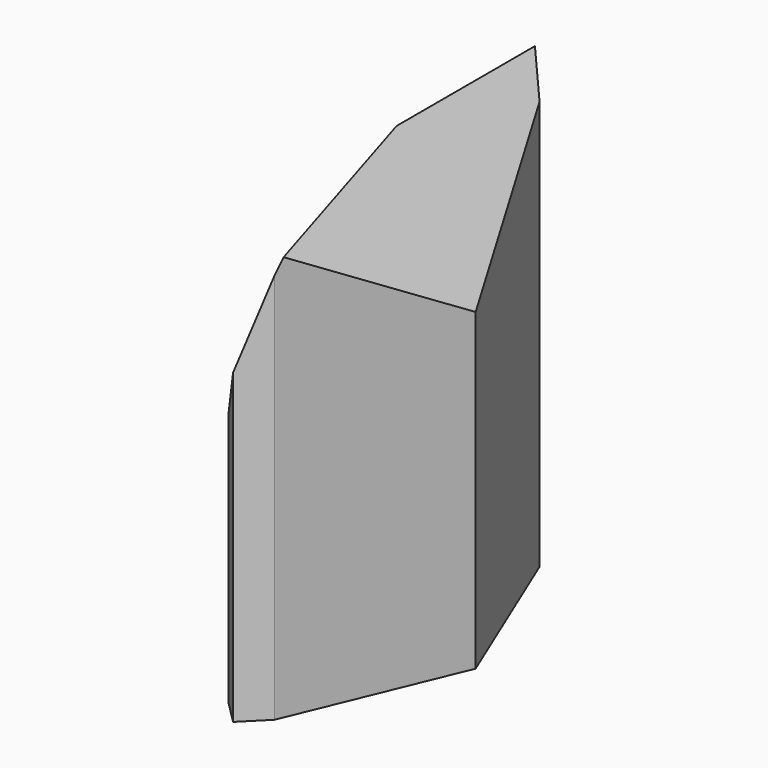
from build123d import *

# Parameters (mm, degrees)
F0_W        = 8.89
F0_H        = 15.24
F1_DEPTH    = 10.16
F3_DEPTH    = 15.24
F4_T1_DEPTH = 36.2882991577
F5_T1_DEPTH = 36.5015311919
F6_T1_DEPTH = 33.8737387742


# Not quite as in the source:
# - a fillet or chamfer that OpenCascade refuses, or shapes differently, is made with other operations: its cross-section is extruded or revolved along the edge and cut away or added


with BuildPart() as f1:
    # F0 (on Top) → F1 (new body)
    with BuildSketch(Plane.XY):
        with Locations((-39.3944829702, 14.0595820769)):
            Rectangle(F0_W, F0_H)
    extrude(amount=F1_DEPTH)

    # F2 (on face) → F3 (join)
    with BuildSketch(Plane.XZ.offset(-6.4395820769)):
        Polygon((-43.8394829702, 10.16), (-34.9494829702, 10.16), (-39.3944829702, 16.349214409), align=None)
    extrude(amount=-F3_DEPTH)

    # F4: chamfer of 5.08 on 4 edges, made by hand

    # F4_s2 → F4_t1 (cut)
    with BuildSketch(Plane.XY.offset(-13.0641495789)):
        Polygon((-34.9494829702, 11.5195820769), (-40.0294829702, 6.4395820769), (-34.9494829702, 6.4395820769), align=None)
        Polygon((-43.8394829702, 11.5195820769), (-38.7594829702, 6.4395820769), (-43.8394829702, 6.4395820769), align=None)
        Polygon((-40.0294829702, 21.6795820769), (-34.9494829702, 16.5995820769), (-34.9494829702, 21.6795820769), align=None)
        Polygon((-38.7594829702, 21.6795820769), (-43.8394829702, 16.5995820769), (-43.8394829702, 21.6795820769), align=None)
    extrude(amount=F4_T1_DEPTH, mode=Mode.SUBTRACT)

    # F5: chamfer of 5.08 on 4 edges, made by hand

    # F5_s2 → F5_t1 (cut)
    with BuildSketch(Plane.XY.offset(-13.170765596)):
        Polygon((-34.9494829702, 11.5195820769), (-38.5415854186, 20.1916845253), (-34.9494829702, 16.5995820769), align=None)
        Polygon((-34.9494829702, 16.5995820769), (-38.5415854186, 7.9274796285), (-34.9494829702, 11.5195820769), align=None)
        Polygon((-40.2473805218, 7.9274796285), (-43.8394829702, 16.5995820769), (-43.8394829702, 11.5195820769), align=None)
        Polygon((-43.8394829702, 11.5195820769), (-40.2473805218, 20.1916845253), (-43.8394829702, 16.5995820769), align=None)
    extrude(amount=F5_T1_DEPTH, mode=Mode.SUBTRACT)

    # F6: chamfer of 5.08 on 1 edges, made by hand

    # F6_s2 → F6_t1 (cut)
    with BuildSketch(Plane(origin=(-11.3557841109, 27.415288012, -15.8117846218), x_dir=(0.9238795325, 0.3826834324, 0), z_dir=(0.3377298738, -0.8153520418, 0.4702548035))):
        Polygon((-34.1500159871, 18.9876434675), (-30.7922479627, 27.8797024774), (-34.1500159871, 24.0676434675), align=None)
    extrude(amount=F6_T1_DEPTH, mode=Mode.SUBTRACT)


solid = f1.part
